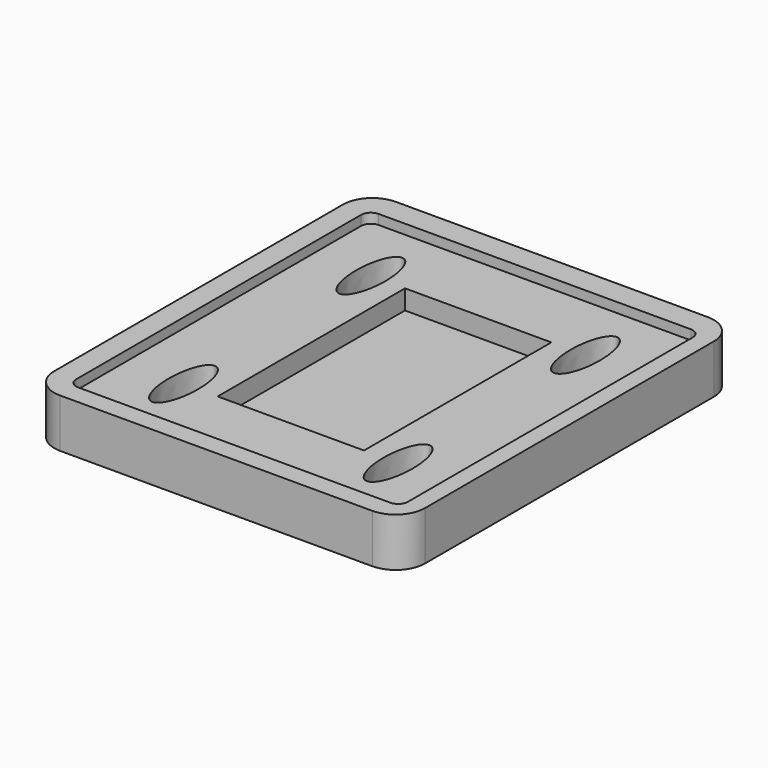
from build123d import *

# Parameters (mm, degrees)
F0_W     = 38
F0_H     = 43
F1_DEPTH = 5
F2_W     = 34
F2_H     = 38.5
F3_DEPTH = 1
F5_DEPTH = 25
F6_R     = 3
F7_R     = 1
F4_W     = 15
F4_H     = 24
F8_DEPTH = 2


# Not quite as in the source:
# - a feature names something its author has since deleted; it is built from what else it names


with BuildPart() as f1:
    # F0 (on Top) → F1 (new body)
    with BuildSketch(Plane.XY):
        with Locations((19, 21.5)):
            Rectangle(F0_W, F0_H)
    extrude(amount=F1_DEPTH)

    # F2 (on face) → F3 (cut)
    with BuildSketch(Plane.XY.offset(5)):
        with Locations((19.25, 21.25)):
            Rectangle(F2_W, F2_H)
    extrude(amount=-F3_DEPTH, mode=Mode.SUBTRACT)

    # F4 (on face) → F5 (cut)
    with BuildSketch(Plane.XY.offset(4)):
        with BuildLine():
            add(Edge.make_bspline(
                [(8.25, 37.25), (5.6519237886, 37.25), (6.9509618943, 31.25), (8.25, 25.25), (9.5490381057, 31.25), (10.8480762114, 37.25), (8.25, 37.25)],
                knots=[0, 0, 0, 2.0943951024, 2.0943951024, 4.1887902048, 4.1887902048, 6.2831853072, 6.2831853072, 6.2831853072], degree=2, weights=[1, 0.5, 1, 0.5, 1, 0.5, 1]))
        make_face()
        with BuildLine():
            add(Edge.make_bspline(
                [(30.25, 37.25), (27.6519237886, 37.25), (28.9509618943, 31.25), (30.25, 25.25), (31.5490381057, 31.25), (32.8480762114, 37.25), (30.25, 37.25)],
                knots=[0, 0, 0, 2.0943951024, 2.0943951024, 4.1887902048, 4.1887902048, 6.2831853072, 6.2831853072, 6.2831853072], degree=2, weights=[1, 0.5, 1, 0.5, 1, 0.5, 1]))
        make_face()
        with BuildLine():
            add(Edge.make_bspline(
                [(30.25, 13.25), (27.6519237886, 13.25), (28.9509618943, 7.25), (30.25, 1.25), (31.5490381057, 7.25), (32.8480762114, 13.25), (30.25, 13.25)],
                knots=[0, 0, 0, 2.0943951024, 2.0943951024, 4.1887902048, 4.1887902048, 6.2831853072, 6.2831853072, 6.2831853072], degree=2, weights=[1, 0.5, 1, 0.5, 1, 0.5, 1]))
        make_face()
        with BuildLine():
            add(Edge.make_bspline(
                [(8.25, 13.25), (5.6519237886, 13.25), (6.9509618943, 7.25), (8.25, 1.25), (9.5490381057, 7.25), (10.8480762114, 13.25), (8.25, 13.25)],
                knots=[0, 0, 0, 2.0943951024, 2.0943951024, 4.1887902048, 4.1887902048, 6.2831853072, 6.2831853072, 6.2831853072], degree=2, weights=[1, 0.5, 1, 0.5, 1, 0.5, 1]))
        make_face()
    extrude(amount=-F5_DEPTH, mode=Mode.SUBTRACT)

    # F6
    f6_edges = [f1.edges().sort_by_distance(p)[0] for p in [
        (0, 0, 2.5),
        (38, 0, 2.5),
        (0, 43, 2.5),
        (38, 43, 2.5),
    ]]
    fillet(f6_edges, radius=F6_R)

    # F7
    f7_edges = [f1.edges().sort_by_distance(p)[0] for p in [
        (2.25, 2, 4.5),
        (2.25, 40.5, 4.5),
        (36.25, 2, 4.5),
        (36.25, 40.5, 4.5),
    ]]
    fillet(f7_edges, radius=F7_R)

    # F4 (on face) → F8 (cut)
    with BuildSketch(Plane.XY.offset(4)):
        with Locations((19.25, 21.25)):
            Rectangle(F4_W, F4_H)
    extrude(amount=-F8_DEPTH, mode=Mode.SUBTRACT)


solid = f1.part
